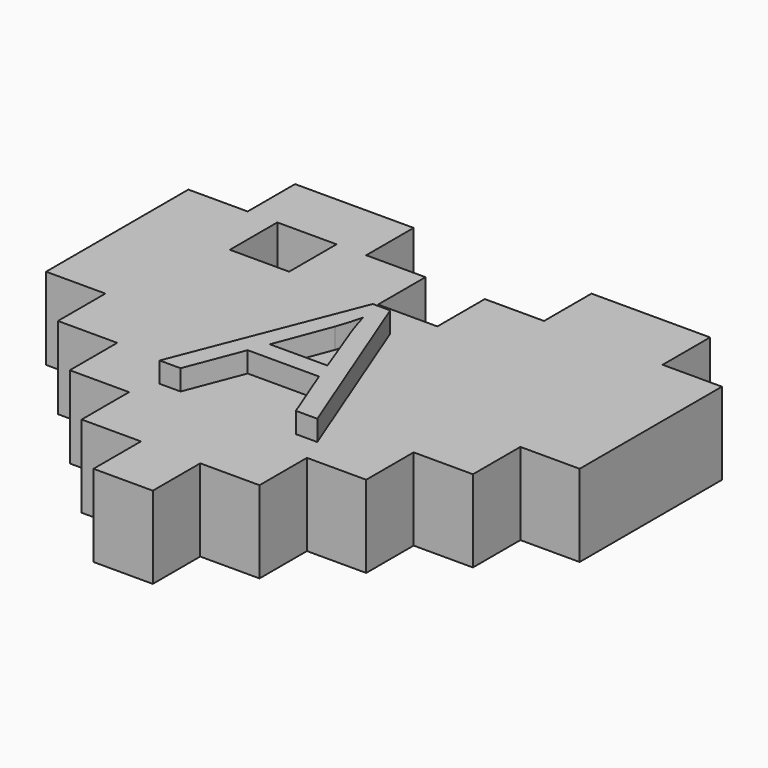
from build123d import *

# Parameters (mm, degrees)
F0_W         = 2.8886614173
F0_H         = 2.8886614173
F1_DEPTH     = 4
F2_TEXT_SIZE = 12.1393072833
F3_DEPTH     = 5


# Not quite as in the source:
# - a feature names something its author has since deleted; it is built from what else it names
# - Text() gives the source's letters only with a copy of the font that has no kerning and outlines rounded to 1/6400 em; it was checked with that copy


with BuildPart() as f1:
    # F0 (on Top) → F1 (new body)
    with BuildSketch(Plane.XY):
        Polygon((-13, 8.6666666667), (-13, 0), (-10.1113385827, 0), (-10.1113385827, -2.8886614173), (-7.2219947507, -2.8886614173), (-7.2219947507, -5.7780052493), (-4.3333333333, -5.7780052493), (-4.3333333333, -8.6666666667), (-1.444671916, -8.6666666667), (-1.444671916, -11.555328084), (1.444671916, -11.555328084), (1.444671916, -8.6666666667), (4.3333333333, -8.6666666667), (4.3333333333, -5.7780052493), (7.2219947507, -5.7780052493), (7.2219947507, -2.8886614173), (10.1113385827, -2.8886614173), (10.1113385827, 0), (13, 0), (13, 8.6666666667), (10.1113385827, 8.6666666667), (10.1113385827, 11.555328084), (4.3333333333, 11.555328084), (4.3333333333, 8.6666666667), (1.444671916, 8.6666666667), (1.444671916, 5.7780052493), (-1.444671916, 5.7780052493), (-1.444671916, 8.6666666667), (-4.3333333333, 8.6666666667), (-4.3333333333, 11.555328084), (-10.1113385827, 11.555328084), (-10.1113385827, 8.6666666667), align=None)
        with Locations((-7.222335958, 7.222335958)):
            Rectangle(F0_W, F0_H, mode=Mode.SUBTRACT)
    extrude(amount=F1_DEPTH)

    # F2 (on face) → F3 (join)
    with BuildSketch(Plane.XY):
        with Locations((-3.8549555466, -4.5152222738)):
            Text('A', F2_TEXT_SIZE, font='Open Sans', text_align=(TextAlign.LEFT, TextAlign.BOTTOM))
    extrude(amount=F3_DEPTH)


solid = f1.part
